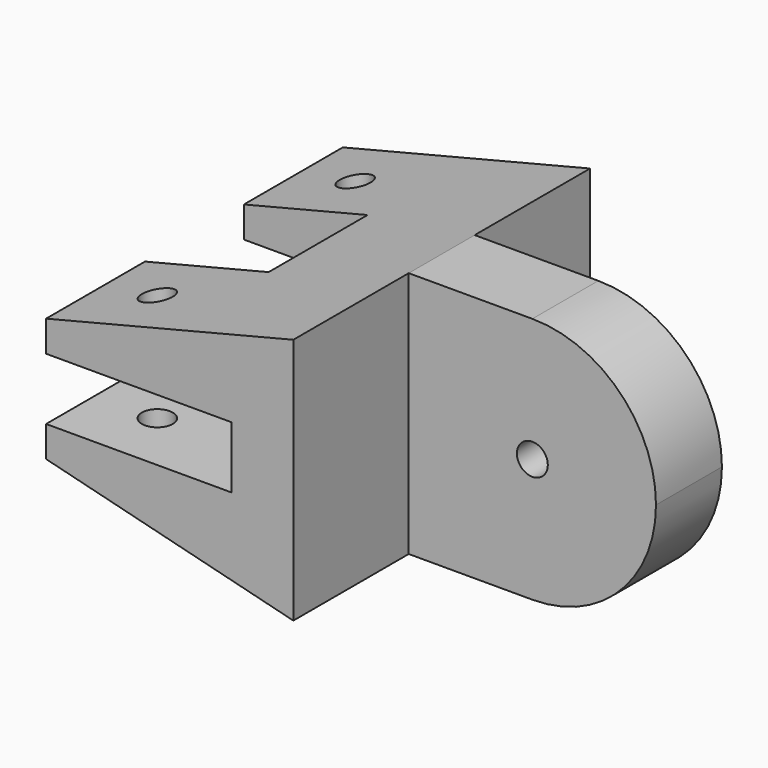
from build123d import *

# Parameters (mm, degrees)
F0_W      = 50.8
F0_H      = 16.9333164
F1_DEPTH  = 50.8
F2_R      = 25.39999
F4_DEPTH  = 119.50414
F5_R      = 3.175
F6_DEPTH  = 61.82298
F7_R      = 3.175
F8_DEPTH  = 63.51287
F9_W      = 38.1
F9_H      = 12.7
F10_DEPTH = 114.99064


# Not quite as in the source:
# - a fillet or chamfer is up to 0.001 mm smaller than in the source, because OpenCascade refuses the exact size


with BuildPart() as f1:
    # F0 (on Top) → F1 (new body)
    with BuildSketch(Plane.XY):
        Polygon((-50.8, 0), (0, 0), (0, 29.633350436), (0, 46.566666836), (0, 76.2), (-50.8, 76.2), (-50.8, 50.8), (-25.4, 50.8), (-25.4, 25.4), (-50.8, 25.4), align=None)
        with Locations((25.4, 38.100008636)):
            Rectangle(F0_W, F0_H)
    extrude(amount=F1_DEPTH)

    # F2 (radius 25.4 in the source; OpenCascade refuses exactly that, so slightly less here)
    f2_edges = [f1.edges().sort_by_distance(p)[0] for p in [
        (50.8, 38.100009, 50.8),
        (50.8, 38.100009, 0),
    ]]
    fillet(f2_edges, radius=F2_R)

    # F3 (on face) → F4 (cut)
    with BuildSketch(Plane.XZ):
        Polygon((-50.8, 50.8), (-50.8, 38.1), (0, 50.8), align=None)
        Polygon((0, 0), (-50.8, 12.7), (-50.8, 0), align=None)
    extrude(amount=-F4_DEPTH, mode=Mode.SUBTRACT)

    # F5 (on face) → F6 (cut)
    with BuildSketch(Plane.XZ.offset(-29.633350436)):
        with Locations((25.4, 25.4)):
            Circle(F5_R)
    extrude(amount=-F6_DEPTH, mode=Mode.SUBTRACT)

    # F7 (on face) → F8 (cut)
    with BuildSketch(Plane.XY):
        with Locations((-38.1, 12.7)):
            Circle(F7_R)
        with Locations((-38.1, 63.5)):
            Circle(F7_R)
    extrude(amount=F8_DEPTH, mode=Mode.SUBTRACT)

    # F9 (on face) → F10 (cut)
    with BuildSketch(Plane.XZ):
        with Locations((-31.75, 25.4)):
            Rectangle(F9_W, F9_H)
    extrude(amount=-F10_DEPTH, mode=Mode.SUBTRACT)


solid = f1.part
